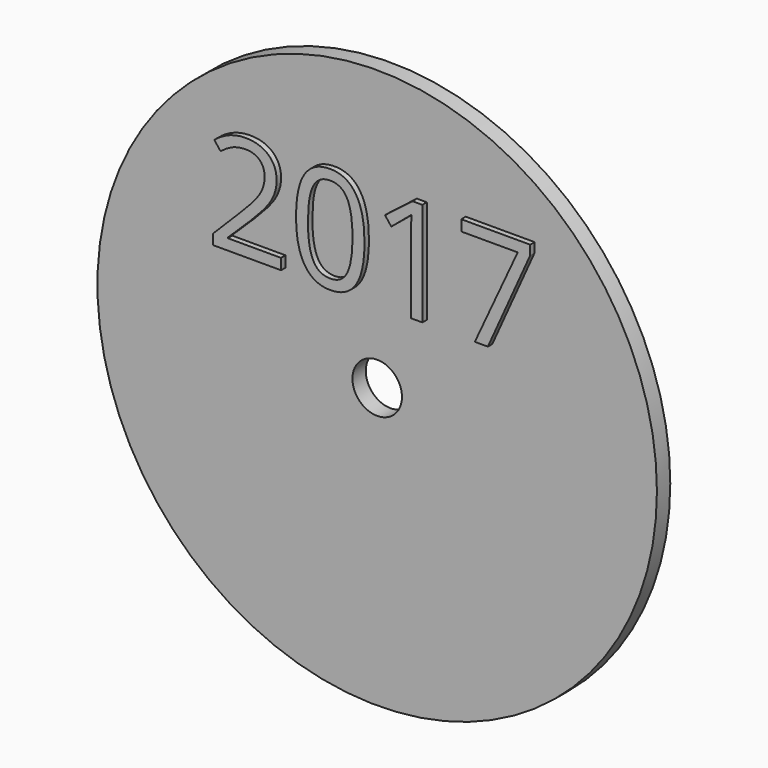
from build123d import *

# Parameters (mm, degrees)
F0_R         = 50.3
F1_DEPTH     = 3
F2_R         = 4.45
F3_DEPTH     = 25
F4_TEXT_SIZE = 26.0763275839
F5_DEPTH     = 1


# Not quite as in the source:
# - Text() gives the source's letters only with a copy of the font that has no kerning and outlines rounded to 1/6400 em; it was checked with that copy


with BuildPart() as f1:
    # F0 (on Front) → F1 (new body)
    with BuildSketch(Plane.XZ):
        Circle(F0_R)
    extrude(amount=F1_DEPTH)

    # F2 (on face) → F3 (cut)
    with BuildSketch(Plane.XZ.offset(3)):
        Circle(F2_R)
    extrude(amount=-F3_DEPTH, mode=Mode.SUBTRACT)

    # F4 (on face) → F5 (join)
    with BuildSketch(Plane.XZ.offset(3)):
        with Locations((-30, 13.6545135119)):
            Text('2017', F4_TEXT_SIZE, font='Open Sans', text_align=(TextAlign.LEFT, TextAlign.BOTTOM))
    extrude(amount=F5_DEPTH)


solid = f1.part
